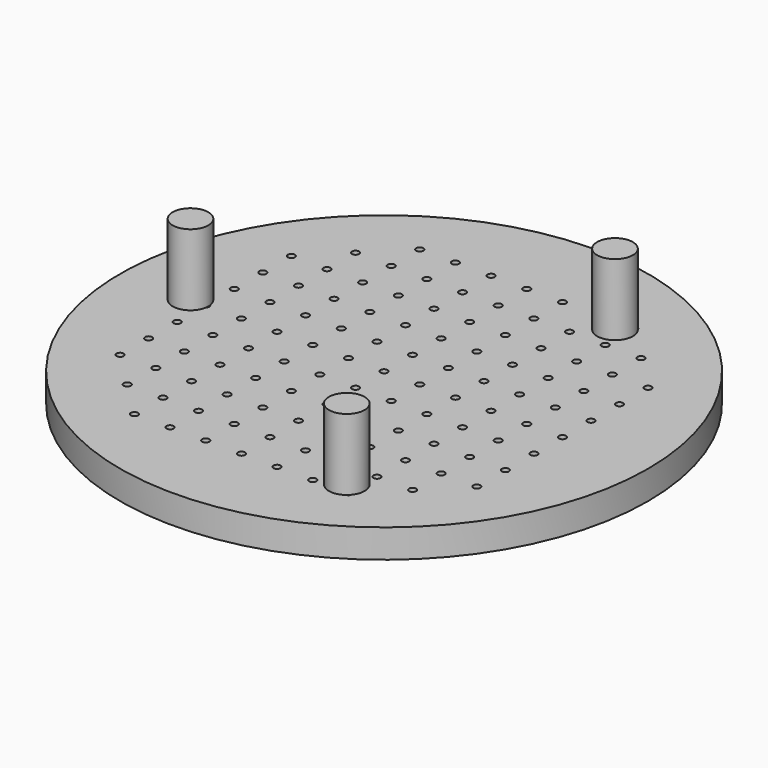
from build123d import *

# Parameters (mm, degrees)
F0_R     = 185
F1_DEPTH = 20
F4_R     = 2.5
F5_DEPTH = 5
F6_R     = 12.5
F7_DEPTH = 50


# Not quite as in the source:
# - the program builds the solid bodies; features that only make, move or delete a surface that nothing else refers to are left out


with BuildPart() as f1:
    # F0 (on Top) → F1 (new body)
    with BuildSketch(Plane.XY):
        Circle(F0_R)
    extrude(amount=F1_DEPTH)

    # F4 (on face) → F5 (cut)
    with BuildSketch(Plane.XY.offset(20)):
        Circle(F4_R)
        with Locations((0, 25)):
            Circle(F4_R)
        with Locations((0, 50)):
            Circle(F4_R)
        with Locations((0, 75)):
            Circle(F4_R)
        with Locations((0, 100)):
            Circle(F4_R)
        with Locations((0, 125)):
            Circle(F4_R)
        with Locations((25, 0)):
            Circle(F4_R)
        with Locations((25, 25)):
            Circle(F4_R)
        with Locations((25, 50)):
            Circle(F4_R)
        with Locations((25, 75)):
            Circle(F4_R)
        with Locations((25, 100)):
            Circle(F4_R)
        with Locations((25, 125)):
            Circle(F4_R)
        with Locations((50, 0)):
            Circle(F4_R)
        with Locations((50, 25)):
            Circle(F4_R)
        with Locations((50, 50)):
            Circle(F4_R)
        with Locations((50, 75)):
            Circle(F4_R)
        with Locations((50, 100)):
            Circle(F4_R)
        with Locations((50, 125)):
            Circle(F4_R)
        with Locations((75, 0)):
            Circle(F4_R)
        with Locations((75, 25)):
            Circle(F4_R)
        with Locations((75, 50)):
            Circle(F4_R)
        with Locations((75, 75)):
            Circle(F4_R)
        with Locations((75, 100)):
            Circle(F4_R)
        with Locations((75, 125)):
            Circle(F4_R)
        with Locations((100, 0)):
            Circle(F4_R)
        with Locations((100, 25)):
            Circle(F4_R)
        with Locations((100, 50)):
            Circle(F4_R)
        with Locations((100, 75)):
            Circle(F4_R)
        with Locations((100, 100)):
            Circle(F4_R)
        with Locations((125, 0)):
            Circle(F4_R)
        with Locations((125, 25)):
            Circle(F4_R)
        with Locations((125, 50)):
            Circle(F4_R)
        with Locations((125, 75)):
            Circle(F4_R)
        with Locations((75, -25)):
            Circle(F4_R)
        with Locations((100, -50)):
            Circle(F4_R)
        with Locations((0, -100)):
            Circle(F4_R)
        with Locations((100, -100)):
            Circle(F4_R)
        with Locations((75, -100)):
            Circle(F4_R)
        with Locations((125, -50)):
            Circle(F4_R)
        with Locations((75, -125)):
            Circle(F4_R)
        with Locations((25, -50)):
            Circle(F4_R)
        with Locations((0, -75)):
            Circle(F4_R)
        with Locations((100, -75)):
            Circle(F4_R)
        with Locations((100, -25)):
            Circle(F4_R)
        with Locations((50, -125)):
            Circle(F4_R)
        with Locations((125, -25)):
            Circle(F4_R)
        with Locations((50, -75)):
            Circle(F4_R)
        with Locations((25, -25)):
            Circle(F4_R)
        with Locations((75, -75)):
            Circle(F4_R)
        with Locations((75, -50)):
            Circle(F4_R)
        with Locations((125, -75)):
            Circle(F4_R)
        with Locations((0, -125)):
            Circle(F4_R)
        with Locations((25, -75)):
            Circle(F4_R)
        with Locations((50, -100)):
            Circle(F4_R)
        with Locations((25, -125)):
            Circle(F4_R)
        with Locations((0, -50)):
            Circle(F4_R)
        with Locations((25, -100)):
            Circle(F4_R)
        with Locations((50, -25)):
            Circle(F4_R)
        with Locations((50, -50)):
            Circle(F4_R)
        with Locations((0, -25)):
            Circle(F4_R)
        with Locations((-25, -75)):
            Circle(F4_R)
        with Locations((-50, -100)):
            Circle(F4_R)
        with Locations((-100, 0)):
            Circle(F4_R)
        with Locations((-100, -100)):
            Circle(F4_R)
        with Locations((-100, -75)):
            Circle(F4_R)
        with Locations((-50, -125)):
            Circle(F4_R)
        with Locations((-125, -75)):
            Circle(F4_R)
        with Locations((-50, -25)):
            Circle(F4_R)
        with Locations((-75, 0)):
            Circle(F4_R)
        with Locations((-75, -100)):
            Circle(F4_R)
        with Locations((-25, -100)):
            Circle(F4_R)
        with Locations((-125, -50)):
            Circle(F4_R)
        with Locations((-25, -125)):
            Circle(F4_R)
        with Locations((-75, -50)):
            Circle(F4_R)
        with Locations((-25, -25)):
            Circle(F4_R)
        with Locations((-75, -75)):
            Circle(F4_R)
        with Locations((-50, -75)):
            Circle(F4_R)
        with Locations((-75, -125)):
            Circle(F4_R)
        with Locations((-125, 0)):
            Circle(F4_R)
        with Locations((-75, -25)):
            Circle(F4_R)
        with Locations((-100, -50)):
            Circle(F4_R)
        with Locations((-125, -25)):
            Circle(F4_R)
        with Locations((-50, 0)):
            Circle(F4_R)
        with Locations((-100, -25)):
            Circle(F4_R)
        with Locations((-25, -50)):
            Circle(F4_R)
        with Locations((-50, -50)):
            Circle(F4_R)
        with Locations((-25, 0)):
            Circle(F4_R)
        with Locations((-75, 25)):
            Circle(F4_R)
        with Locations((-100, 50)):
            Circle(F4_R)
        with Locations((-100, 100)):
            Circle(F4_R)
        with Locations((-75, 100)):
            Circle(F4_R)
        with Locations((-125, 50)):
            Circle(F4_R)
        with Locations((-75, 125)):
            Circle(F4_R)
        with Locations((-25, 50)):
            Circle(F4_R)
        with Locations((-100, 75)):
            Circle(F4_R)
        with Locations((-100, 25)):
            Circle(F4_R)
        with Locations((-50, 125)):
            Circle(F4_R)
        with Locations((-125, 25)):
            Circle(F4_R)
        with Locations((-50, 75)):
            Circle(F4_R)
        with Locations((-25, 25)):
            Circle(F4_R)
        with Locations((-75, 75)):
            Circle(F4_R)
        with Locations((-75, 50)):
            Circle(F4_R)
        with Locations((-125, 75)):
            Circle(F4_R)
        with Locations((-25, 75)):
            Circle(F4_R)
        with Locations((-50, 100)):
            Circle(F4_R)
        with Locations((-25, 125)):
            Circle(F4_R)
        with Locations((-25, 100)):
            Circle(F4_R)
        with Locations((-50, 25)):
            Circle(F4_R)
        with Locations((-50, 50)):
            Circle(F4_R)
    extrude(amount=-F5_DEPTH, mode=Mode.SUBTRACT)

    # F6 (on face) → F7 (join)
    with BuildSketch(Plane.XY.offset(20)):
        with Locations((-135.6773132596, 0)):
            Circle(F6_R)
        with Locations((67.8386566298, -117.5)):
            Circle(F6_R)
        with Locations((67.8386566298, 117.5)):
            Circle(F6_R)
    extrude(amount=F7_DEPTH)


solid = f1.part
